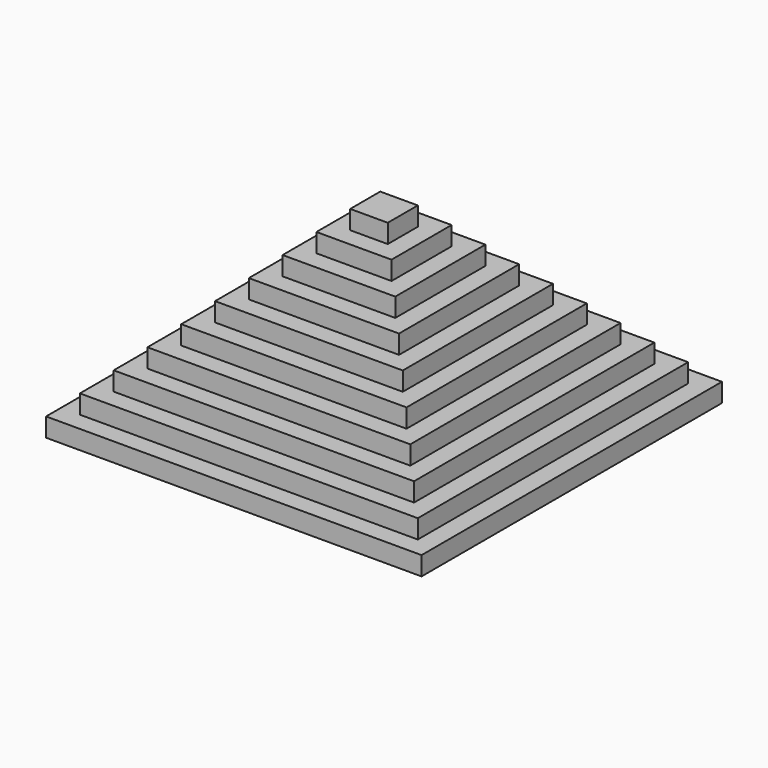
from build123d import *

# Parameters (mm, degrees)
F0_W      = 100
F0_H      = 100
F1_DEPTH  = 5
F2_W      = 95
F2_H      = 95
F3_DEPTH  = 3
F4_W      = 95
F4_H      = 95
F5_DEPTH  = 2
F6_W      = 95
F6_H      = 95
F7_DEPTH  = 1
F8_W      = 90
F8_H      = 90
F9_DEPTH  = 5
F10_W     = 85
F10_H     = 85
F11_DEPTH = 3
F12_W     = 85
F12_H     = 85
F13_DEPTH = 2
F14_W     = 85
F14_H     = 85
F15_DEPTH = 1
F16_W     = 80
F16_H     = 80
F17_DEPTH = 5
F18_W     = 75
F18_H     = 75
F19_DEPTH = 3
F20_W     = 75
F20_H     = 75
F21_DEPTH = 2
F22_W     = 75
F22_H     = 75
F23_DEPTH = 1
F24_W     = 70
F24_H     = 70
F25_DEPTH = 5
F26_W     = 65
F26_H     = 65
F27_DEPTH = 3
F28_W     = 65
F28_H     = 65
F29_DEPTH = 2
F30_W     = 65
F30_H     = 65
F31_DEPTH = 1
F32_W     = 60
F32_H     = 60
F33_DEPTH = 5
F34_W     = 55
F34_H     = 55
F35_DEPTH = 3
F36_W     = 55
F36_H     = 55
F37_DEPTH = 2
F38_W     = 55
F38_H     = 55
F39_DEPTH = 1
F40_W     = 50
F40_H     = 50
F41_DEPTH = 5
F42_W     = 45
F42_H     = 45
F43_DEPTH = 3
F44_W     = 45
F44_H     = 45
F45_DEPTH = 2
F46_W     = 45
F46_H     = 45
F47_DEPTH = 1
F48_W     = 40
F48_H     = 40
F49_DEPTH = 5
F50_W     = 35
F50_H     = 35
F51_DEPTH = 3
F52_W     = 35
F52_H     = 35
F53_DEPTH = 2
F54_W     = 35
F54_H     = 35
F55_DEPTH = 1
F56_W     = 30
F56_H     = 30
F57_DEPTH = 5
F58_W     = 25
F58_H     = 25
F59_DEPTH = 3
F60_W     = 25
F60_H     = 25
F61_DEPTH = 2
F62_W     = 25
F62_H     = 25
F63_DEPTH = 1
F64_W     = 20
F64_H     = 20
F65_DEPTH = 5
F66_W     = 15
F66_H     = 15
F67_DEPTH = 3
F68_W     = 15
F68_H     = 15
F69_DEPTH = 2
F70_W     = 15
F70_H     = 15
F71_DEPTH = 1
F72_W     = 10
F72_H     = 10
F73_DEPTH = 5
F74_W     = 5
F74_H     = 5
F75_DEPTH = 3
F76_W     = 5
F76_H     = 5
F77_DEPTH = 2
F78_W     = 5
F78_H     = 5
F79_DEPTH = 1


with BuildPart() as f1:
    # F0 (on Top) → F1 (new body)
    with BuildSketch(Plane.XY):
        Rectangle(F0_W, F0_H)
    extrude(amount=F1_DEPTH)

    # F2 (on face) → F3 (cut)
    with BuildSketch(Plane.XY.offset(5)):
        Rectangle(F2_W, F2_H)
    extrude(amount=-F3_DEPTH, mode=Mode.SUBTRACT)

    # F6 (on face) → F7 (join)
    with BuildSketch(Plane.XY.offset(4)):
        Rectangle(F6_W, F6_H)
    extrude(amount=F7_DEPTH)

    # F8 (on face) → F9 (join)
    with BuildSketch(Plane.XY.offset(5)):
        Rectangle(F8_W, F8_H)
    extrude(amount=F9_DEPTH)

    # F10 (on face) → F11 (cut)
    with BuildSketch(Plane.XY.offset(10)):
        Rectangle(F10_W, F10_H)
    extrude(amount=-F11_DEPTH, mode=Mode.SUBTRACT)

    # F14 (on face) → F15 (join)
    with BuildSketch(Plane.XY.offset(9)):
        Rectangle(F14_W, F14_H)
    extrude(amount=F15_DEPTH)

    # F16 (on face) → F17 (join)
    with BuildSketch(Plane.XY.offset(10)):
        Rectangle(F16_W, F16_H)
    extrude(amount=F17_DEPTH)

    # F18 (on face) → F19 (cut)
    with BuildSketch(Plane.XY.offset(15)):
        Rectangle(F18_W, F18_H)
    extrude(amount=-F19_DEPTH, mode=Mode.SUBTRACT)

    # F22 (on face) → F23 (join)
    with BuildSketch(Plane.XY.offset(14)):
        Rectangle(F22_W, F22_H)
    extrude(amount=F23_DEPTH)

    # F24 (on face) → F25 (join)
    with BuildSketch(Plane.XY.offset(15)):
        Rectangle(F24_W, F24_H)
    extrude(amount=F25_DEPTH)

    # F26 (on face) → F27 (cut)
    with BuildSketch(Plane.XY.offset(20)):
        Rectangle(F26_W, F26_H)
    extrude(amount=-F27_DEPTH, mode=Mode.SUBTRACT)

    # F30 (on face) → F31 (join)
    with BuildSketch(Plane.XY.offset(19)):
        Rectangle(F30_W, F30_H)
    extrude(amount=F31_DEPTH)

    # F32 (on face) → F33 (join)
    with BuildSketch(Plane.XY.offset(20)):
        Rectangle(F32_W, F32_H)
    extrude(amount=F33_DEPTH)

    # F34 (on face) → F35 (cut)
    with BuildSketch(Plane.XY.offset(25)):
        Rectangle(F34_W, F34_H)
    extrude(amount=-F35_DEPTH, mode=Mode.SUBTRACT)

    # F38 (on face) → F39 (join)
    with BuildSketch(Plane.XY.offset(24)):
        Rectangle(F38_W, F38_H)
    extrude(amount=F39_DEPTH)

    # F40 (on face) → F41 (join)
    with BuildSketch(Plane.XY.offset(25)):
        Rectangle(F40_W, F40_H)
    extrude(amount=F41_DEPTH)

    # F42 (on face) → F43 (cut)
    with BuildSketch(Plane.XY.offset(30)):
        Rectangle(F42_W, F42_H)
    extrude(amount=-F43_DEPTH, mode=Mode.SUBTRACT)

    # F46 (on face) → F47 (join)
    with BuildSketch(Plane.XY.offset(29)):
        Rectangle(F46_W, F46_H)
    extrude(amount=F47_DEPTH)

    # F48 (on face) → F49 (join)
    with BuildSketch(Plane.XY.offset(30)):
        Rectangle(F48_W, F48_H)
    extrude(amount=F49_DEPTH)

    # F50 (on face) → F51 (cut)
    with BuildSketch(Plane.XY.offset(35)):
        Rectangle(F50_W, F50_H)
    extrude(amount=-F51_DEPTH, mode=Mode.SUBTRACT)

    # F54 (on face) → F55 (join)
    with BuildSketch(Plane.XY.offset(34)):
        Rectangle(F54_W, F54_H)
    extrude(amount=F55_DEPTH)

    # F56 (on face) → F57 (join)
    with BuildSketch(Plane.XY.offset(35)):
        Rectangle(F56_W, F56_H)
    extrude(amount=F57_DEPTH)

    # F58 (on face) → F59 (cut)
    with BuildSketch(Plane.XY.offset(40)):
        Rectangle(F58_W, F58_H)
    extrude(amount=-F59_DEPTH, mode=Mode.SUBTRACT)

    # F62 (on face) → F63 (join)
    with BuildSketch(Plane.XY.offset(39)):
        Rectangle(F62_W, F62_H)
    extrude(amount=F63_DEPTH)

    # F64 (on face) → F65 (join)
    with BuildSketch(Plane.XY.offset(40)):
        Rectangle(F64_W, F64_H)
    extrude(amount=F65_DEPTH)

    # F66 (on face) → F67 (cut)
    with BuildSketch(Plane.XY.offset(45)):
        Rectangle(F66_W, F66_H)
    extrude(amount=-F67_DEPTH, mode=Mode.SUBTRACT)

    # F70 (on face) → F71 (join)
    with BuildSketch(Plane.XY.offset(44)):
        Rectangle(F70_W, F70_H)
    extrude(amount=F71_DEPTH)

    # F72 (on face) → F73 (join)
    with BuildSketch(Plane.XY.offset(45)):
        Rectangle(F72_W, F72_H)
    extrude(amount=F73_DEPTH)

    # F74 (on face) → F75 (cut)
    with BuildSketch(Plane.XY.offset(50)):
        Rectangle(F74_W, F74_H)
    extrude(amount=-F75_DEPTH, mode=Mode.SUBTRACT)

    # F78 (on face) → F79 (join)
    with BuildSketch(Plane.XY.offset(49)):
        Rectangle(F78_W, F78_H)
    extrude(amount=F79_DEPTH)


with BuildPart() as f5:
    # F4 (on face) → F5 (new body)
    with BuildSketch(Plane.XY.offset(2)):
        Rectangle(F4_W, F4_H)
    extrude(amount=F5_DEPTH)


with BuildPart() as f13:
    # F12 (on face) → F13 (new body)
    with BuildSketch(Plane.XY.offset(7)):
        Rectangle(F12_W, F12_H)
    extrude(amount=F13_DEPTH)


with BuildPart() as f21:
    # F20 (on face) → F21 (new body)
    with BuildSketch(Plane.XY.offset(12)):
        Rectangle(F20_W, F20_H)
    extrude(amount=F21_DEPTH)


with BuildPart() as f29:
    # F28 (on face) → F29 (new body)
    with BuildSketch(Plane.XY.offset(17)):
        Rectangle(F28_W, F28_H)
    extrude(amount=F29_DEPTH)


with BuildPart() as f37:
    # F36 (on face) → F37 (new body)
    with BuildSketch(Plane.XY.offset(22)):
        Rectangle(F36_W, F36_H)
    extrude(amount=F37_DEPTH)


with BuildPart() as f45:
    # F44 (on face) → F45 (new body)
    with BuildSketch(Plane.XY.offset(27)):
        Rectangle(F44_W, F44_H)
    extrude(amount=F45_DEPTH)


with BuildPart() as f53:
    # F52 (on face) → F53 (new body)
    with BuildSketch(Plane.XY.offset(32)):
        Rectangle(F52_W, F52_H)
    extrude(amount=F53_DEPTH)


with BuildPart() as f61:
    # F60 (on face) → F61 (new body)
    with BuildSketch(Plane.XY.offset(37)):
        Rectangle(F60_W, F60_H)
    extrude(amount=F61_DEPTH)


with BuildPart() as f69:
    # F68 (on face) → F69 (new body)
    with BuildSketch(Plane.XY.offset(42)):
        Rectangle(F68_W, F68_H)
    extrude(amount=F69_DEPTH)


with BuildPart() as f77:
    # F76 (on face) → F77 (new body)
    with BuildSketch(Plane.XY.offset(47)):
        Rectangle(F76_W, F76_H)
    extrude(amount=F77_DEPTH)


solid = Compound([f1.part, f5.part, f13.part, f21.part, f29.part, f37.part, f45.part, f53.part, f61.part, f69.part, f77.part])
